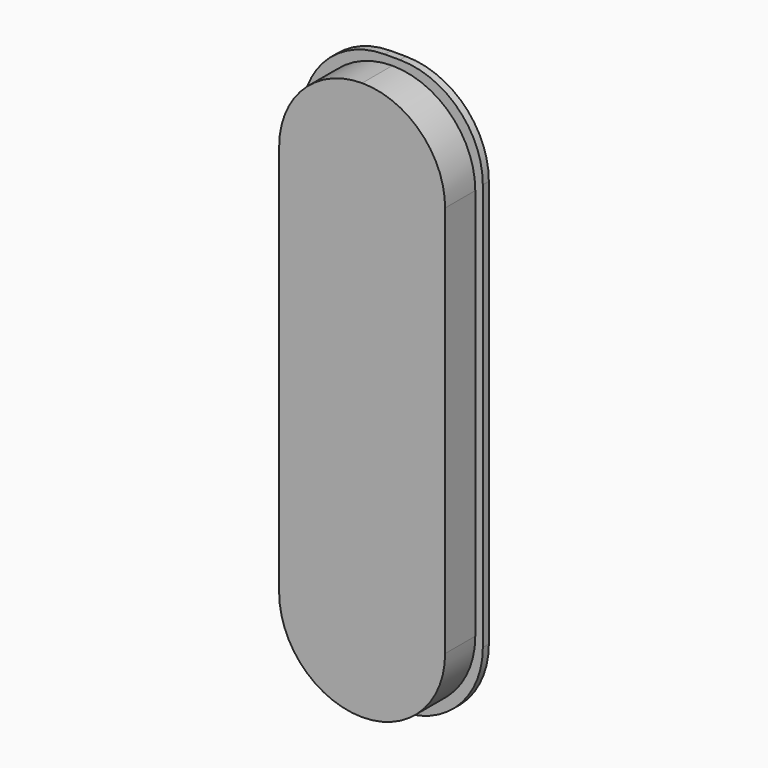
from build123d import *

# Parameters (mm, degrees)
F0_W          = 22
F0_H          = 74
F0_W_2        = 20
F0_H_2        = 72
F1_DEPTH      = 6
F0_W_3        = 24
F0_H_3        = 76
F2_DEPTH      = 1
F3_DEPTH      = 5
F4_F1_R       = 10.9999
F4_F2_R       = 11
F4_2_T1_DEPTH = 5
F4_2_T3_DEPTH = 61


# Not quite as in the source:
# - a fillet or chamfer that OpenCascade refuses, or shapes differently, is made with other operations: its cross-section is extruded or revolved along the edge and cut away or added
# - a fillet or chamfer is up to 0.001 mm smaller than in the source, because OpenCascade refuses the exact size


with BuildPart() as f1:
    # F0 (on Front) → F1 (new body)
    with BuildSketch(Plane.XZ):
        with Locations((10, 15.842890054)):
            Rectangle(F0_W, F0_H)
        with Locations((10, 15.842890054)):
            Rectangle(F0_W_2, F0_H_2, mode=Mode.SUBTRACT)
        with Locations((10, 15.842890054)):
            Rectangle(F0_W_2, F0_H_2)
    extrude(amount=F1_DEPTH)

    # F0 (on Front) → F3 (cut)
    with BuildSketch(Plane.XZ):
        with Locations((10, 15.842890054)):
            Rectangle(F0_W_2, F0_H_2)
    extrude(amount=F3_DEPTH, mode=Mode.SUBTRACT)

    # F4#2: fillet of radius 11 on 8 edges, made by hand

    # F4_2_s2 → F4_2_t1 (join)
    with BuildSketch(Plane.XZ):
        with BuildLine():
            ThreePointArc((20, 40.842890054), (16.7781745931, 48.621064647), (9, 51.842890054))
            Line((9, 51.842890054), (20, 51.842890054))
            Line((20, 51.842890054), (20, 40.842890054))
        make_face()
        with BuildLine():
            ThreePointArc((11, 51.842890054), (3.2218254069, 48.621064647), (0, 40.842890054))
            Line((0, 40.842890054), (0, 51.842890054))
            Line((0, 51.842890054), (11, 51.842890054))
        make_face()
        with BuildLine():
            ThreePointArc((0, -9.157109946), (3.2218254069, -16.9352845391), (11, -20.157109946))
            Line((11, -20.157109946), (0, -20.157109946))
            Line((0, -20.157109946), (0, -9.157109946))
        make_face()
        with BuildLine():
            ThreePointArc((20, -9.157109946), (16.7781745931, -16.9352845391), (9, -20.157109946))
            Line((9, -20.157109946), (20, -20.157109946))
            Line((20, -20.157109946), (20, -9.157109946))
        make_face()
    extrude(amount=F4_2_T1_DEPTH)

    # F4_2_s4 → F4_2_t3 (cut)
    with BuildSketch(Plane.XZ.offset(-27.5)):
        with BuildLine():
            ThreePointArc((21, 41.842890054), (17.7781745931, 49.621064647), (10, 52.842890054))
            Line((10, 52.842890054), (21, 52.842890054))
            Line((21, 52.842890054), (21, 41.842890054))
        make_face()
        with BuildLine():
            ThreePointArc((10, 52.842890054), (2.2218254069, 49.621064647), (-1, 41.842890054))
            Line((-1, 41.842890054), (-1, 52.842890054))
            Line((-1, 52.842890054), (10, 52.842890054))
        make_face()
        with BuildLine():
            ThreePointArc((10, -21.157109946), (2.2218254069, -17.9352845391), (-1, -10.157109946))
            Line((-1, -10.157109946), (-1, -21.157109946))
            Line((-1, -21.157109946), (10, -21.157109946))
        make_face()
        with BuildLine():
            ThreePointArc((21, -10.157109946), (17.7781745931, -17.9352845391), (10, -21.157109946))
            Line((10, -21.157109946), (21, -21.157109946))
            Line((21, -21.157109946), (21, -10.157109946))
        make_face()
    extrude(amount=F4_2_T3_DEPTH, mode=Mode.SUBTRACT)


with BuildPart() as f2:
    # F0 (on Front) → F2 (new body)
    with BuildSketch(Plane.XZ):
        with Locations((10, 15.842890054)):
            Rectangle(F0_W_3, F0_H_3)
        with Locations((10, 15.842890054)):
            Rectangle(F0_W, F0_H, mode=Mode.SUBTRACT)
    extrude(amount=F2_DEPTH)

    # F4: fillet of radius 11 on 8 edges, made by hand

    # F4_f1 (radius 11 in the source; OpenCascade refuses exactly that, so slightly less here)
    f4_f1_edges = [f2.edges().sort_by_distance(p)[0] for p in [
        (21, -0.5, 52.842890054),
        (-1, -0.5, 52.842890054),
        (-1, -0.5, -21.157109946),
        (21, -0.5, -21.157109946),
    ]]
    fillet(f4_f1_edges, radius=F4_F1_R)

    # F4_f2
    f4_f2_edges = [f2.edges().sort_by_distance(p)[0] for p in [
        (22, -0.5, 53.842890054),
        (-2, -0.5, 53.842890054),
        (-2, -0.5, -22.157109946),
        (22, -0.5, -22.157109946),
    ]]
    fillet(f4_f2_edges, radius=F4_F2_R)


solid = Compound([f1.part, f2.part])
